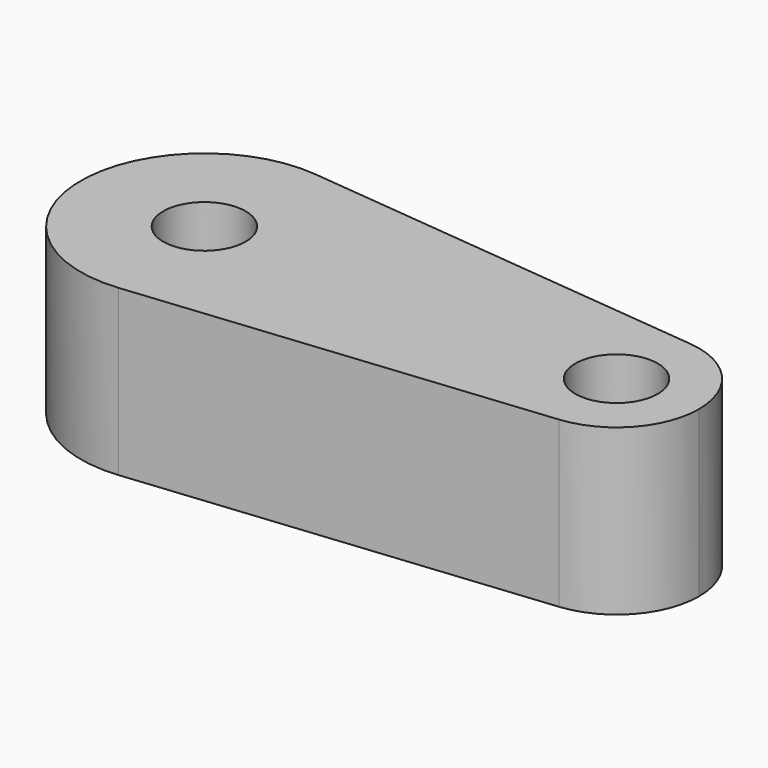
from build123d import *

# Parameters (mm, degrees)
F0_R     = 12.7
F1_DEPTH = 50.8


# Not quite as in the source:
# - the program builds the solid bodies; features that only make, move or delete a surface that nothing else refers to are left out


with BuildPart() as f1:
    # F0 (on Top) → F1 (new body)
    with BuildSketch(Plane.XY):
        with BuildLine():
            ThreePointArc((3.81, -37.9090213538), (28.2557162358, -25.5582569828), (38.1, 0))
            ThreePointArc((38.1, 0), (28.2557162358, 25.5582569828), (3.81, 37.9090213538))
            ThreePointArc((3.81, 37.9090213538), (-38.1, 0), (3.81, -37.9090213538))
        make_face()
        Circle(F0_R, mode=Mode.SUBTRACT)
        with BuildLine():
            ThreePointArc((3.81, 37.9090213538), (28.2557162358, 25.5582569828), (38.1, 0))
            ThreePointArc((38.1, 0), (28.2557162358, -25.5582569828), (3.81, -37.9090213538))
            Line((3.81, -37.9090213538), (129.54, -25.2726809025))
            ThreePointArc((129.54, -25.2726809025), (101.6, 0), (129.54, 25.2726809025))
            Line((129.54, 25.2726809025), (3.81, 37.9090213538))
        make_face()
        with BuildLine():
            ThreePointArc((152.4, 0), (145.8371441572, 17.0388379885), (129.54, 25.2726809025))
            ThreePointArc((129.54, 25.2726809025), (101.6, 0), (129.54, -25.2726809025))
            ThreePointArc((129.54, -25.2726809025), (145.8371441572, -17.0388379885), (152.4, 0))
        make_face()
        with Locations((127, 0)):
            Circle(F0_R, mode=Mode.SUBTRACT)
    extrude(amount=F1_DEPTH)


solid = f1.part
